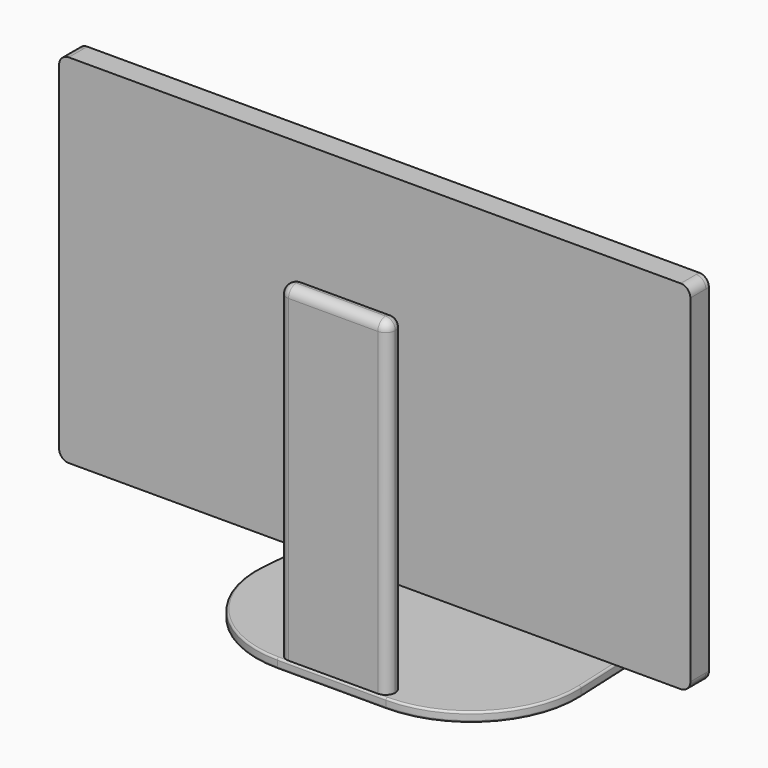
from build123d import *

# Parameters (mm, degrees)
F1_DEPTH    = 5
F2_R        = 1
F3_W        = 56.1862232486
F3_H        = 10
F4_DEPTH    = 170
F5_T1_DEPTH = 170
F6_T1_DEPTH = 170
F8_DEPTH    = 16
F9_R        = 4.99999
F11_DEPTH   = 10
F12_W       = 24
F12_H       = 13.9404982328
F13_DEPTH   = 10
F14_R       = 5
F15_R       = 5
F16_W       = 316.6455233097
F16_H       = 174.8104447126
F17_DEPTH   = 2
F18_W       = 15
F18_H       = 2
F19_DEPTH   = 0.5
F20_R       = 5
F21_R       = 5


# Not quite as in the source:
# - a fillet or chamfer that OpenCascade refuses, or shapes differently, is made with other operations: its cross-section is extruded or revolved along the edge and cut away or added
# - a fillet or chamfer is up to 0.001 mm smaller than in the source, because OpenCascade refuses the exact size


with BuildPart() as f1:
    # F0 (on Top) → F1 (new body)
    with BuildSketch(Plane.XY):
        with BuildLine():
            Line((23.2672947912, 89.7089094173), (-23.969883312, 89.7089094173))
            ThreePointArc((-23.969883312, 89.7089094173), (-61.030315745, 75.3478605341), (-78.737050658, 39.7643402492))
            Line((-78.737050658, 39.7643402492), (-84.7743571616, -25.63981354))
            ThreePointArc((-84.7743571616, -25.63981354), (-70.6461409325, -67.7556768049), (-30.0071898156, -85.6952443719))
            Line((-30.0071898156, -85.6952443719), (26.1790334329, -85.6952443719))
            ThreePointArc((26.1790334329, -85.6952443719), (65.9253366057, -68.7114433416), (81.1246105138, -28.2491128847))
            Line((81.1246105138, -28.2491128847), (78.2128718721, 37.1550409045))
            ThreePointArc((78.2128718721, 37.1550409045), (61.2834937609, 74.45521259), (23.2672947912, 89.7089094173))
        make_face()
    extrude(amount=F1_DEPTH)

    # F2
    f2_edges = [f1.edges().sort_by_distance(p)[0] for p in [
        (79.668741, 4.452964, 0),
        (61.283494, 74.455213, 0),
        (-0.351294, 89.708909, 0),
        (-61.030316, 75.347861, 0),
        (-81.755704, 7.062263, 0),
        (-70.646141, -67.755677, 0),
        (-1.914078, -85.695244, 0),
        (65.925337, -68.711443, 0),
        (79.668741, 4.452964, 5),
        (61.283494, 74.455213, 5),
        (-0.351294, 89.708909, 5),
        (-61.030316, 75.347861, 5),
        (-81.755704, 7.062263, 5),
        (-70.646141, -67.755677, 5),
        (-1.914078, -85.695244, 5),
        (65.925337, -68.711443, 5),
    ]]
    fillet(f2_edges, radius=F2_R)

    # F3 (on face) → F4 (join)
    with BuildSketch(Plane.XY.offset(5)):
        with Locations((-1.9140781913, -79.6952443719)):
            Rectangle(F3_W, F3_H)
    extrude(amount=F4_DEPTH)

    # F5: fillet of radius 5 on 1 edges, made by hand

    # F5_s2 → F5_t1 (cut)
    with BuildSketch(Plane.XY.offset(5)):
        with BuildLine():
            ThreePointArc((26.1790334329, -79.6952443719), (24.7145673389, -83.2307782778), (21.1790334329, -84.6952443719))
            Line((21.1790334329, -84.6952443719), (21.1790334329, -84.7952443719))
            Line((21.1790334329, -84.7952443719), (26.2790334329, -84.7952443719))
            Line((26.2790334329, -84.7952443719), (26.2790334329, -79.6952443719))
            Line((26.2790334329, -79.6952443719), (26.1790334329, -79.6952443719))
        make_face()
    extrude(amount=F5_T1_DEPTH, mode=Mode.SUBTRACT)

    # F6: fillet of radius 5 on 3 edges, made by hand

    # F6_s2 → F6_t1 (cut)
    with BuildSketch(Plane.XY.offset(5)):
        with BuildLine():
            ThreePointArc((21.1790334329, -74.6952443719), (24.7145673389, -76.159710466), (26.1790334329, -79.6952443719))
            Line((26.1790334329, -79.6952443719), (26.2790334329, -79.6952443719))
            Line((26.2790334329, -79.6952443719), (26.2790334329, -74.5952443719))
            Line((26.2790334329, -74.5952443719), (21.1790334329, -74.5952443719))
            Line((21.1790334329, -74.5952443719), (21.1790334329, -74.6952443719))
        make_face()
        with BuildLine():
            ThreePointArc((-25.0071898156, -74.6952443719), (-28.5427237216, -76.159710466), (-30.0071898156, -79.6952443719))
            Line((-30.0071898156, -79.6952443719), (-30.1071898156, -79.6952443719))
            Line((-30.1071898156, -79.6952443719), (-30.1071898156, -74.5952443719))
            Line((-30.1071898156, -74.5952443719), (-25.0071898156, -74.5952443719))
            Line((-25.0071898156, -74.5952443719), (-25.0071898156, -74.6952443719))
        make_face()
        with BuildLine():
            ThreePointArc((-30.0071898156, -79.6952443719), (-28.5427237216, -83.2307782778), (-25.0071898156, -84.6952443719))
            Line((-25.0071898156, -84.6952443719), (-25.0071898156, -84.7952443719))
            Line((-25.0071898156, -84.7952443719), (-30.1071898156, -84.7952443719))
            Line((-30.1071898156, -84.7952443719), (-30.1071898156, -79.6952443719))
            Line((-30.1071898156, -79.6952443719), (-30.0071898156, -79.6952443719))
        make_face()
    extrude(amount=F6_T1_DEPTH, mode=Mode.SUBTRACT)

    # F7 (on face) → F8 (join)
    with BuildSketch(Plane(origin=(0, -74.6952443719, 0), x_dir=(-1, 0, 0), z_dir=(0, 1, 0))):
        Polygon((13.9140781913, 140.0128751993), (1.9140781913, 140.0128751993), (-10.0859218087, 140.0128751993), (-10.0859218087, 126.0723769665), (13.9140781913, 126.0723769665), align=None)
    extrude(amount=F8_DEPTH)

    # F9 (radius 5 in the source; OpenCascade refuses exactly that, so slightly less here)
    f9_edges = [f1.edges().sort_by_distance(p)[0] for p in [
        (-1.914078, -74.695244, 175),
        (-28.542724, -76.15971, 175),
        (24.714567, -76.15971, 175),
        (24.714567, -83.230778, 175),
        (-1.914078, -84.695244, 175),
        (-28.542724, -83.230778, 175),
    ]]
    fillet(f9_edges, radius=F9_R)

    # F20
    f20_edges = [f1.edges().sort_by_distance(p)[0] for p in [
        (-13.914078, -66.695244, 140.012875),
    ]]
    fillet(f20_edges, radius=F20_R)

    # F21
    f21_edges = [f1.edges().sort_by_distance(p)[0] for p in [
        (-13.914078, -66.695244, 126.072377),
        (10.085922, -66.695244, 140.012875),
        (10.085922, -66.695244, 126.072377),
    ]]
    fillet(f21_edges, radius=F21_R)


with BuildPart() as f11:
    # F10 (on face) → F11 (new body)
    with BuildSketch(Plane(origin=(0, -58.6952443719, 0), x_dir=(-1, 0, 0), z_dir=(0, 1, 0))):
        Polygon((164.5585149527, 225.5081981421), (1.9140781913, 225.5081981421), (-162.087008357, 225.5081981421), (-162.087008357, 40.6977534294), (-160.0567102432, 40.6977534294), (164.5585149527, 40.6977534294), align=None)
        Polygon((-10.0859218087, 140.0128751993), (1.9140781913, 140.0128751993), (13.9140781913, 140.0128751993), (13.9140781913, 126.0723769665), (-10.0859218087, 126.0723769665), align=None, mode=Mode.SUBTRACT)
    extrude(amount=F11_DEPTH)

    # F14
    f14_edges = [f11.edges().sort_by_distance(p)[0] for p in [
        (162.087008, -53.695244, 225.508198),
    ]]
    fillet(f14_edges, radius=F14_R)

    # F15
    f15_edges = [f11.edges().sort_by_distance(p)[0] for p in [
        (-164.558515, -53.695244, 225.508198),
        (-164.558515, -53.695244, 40.697753),
        (162.087008, -53.695244, 40.697753),
    ]]
    fillet(f15_edges, radius=F15_R)

    # F16 (on face) → F17 (join)
    with BuildSketch(Plane(origin=(0, -48.6952443719, 0), x_dir=(-1, 0, 0), z_dir=(0, 1, 0))):
        with BuildLine():
            ThreePointArc((164.5585149527, 220.5081981421), (163.0940488586, 224.043732048), (159.5585149527, 225.5081981421))
            Line((159.5585149527, 225.5081981421), (-157.087008357, 225.5081981421))
            ThreePointArc((-157.087008357, 225.5081981421), (-160.622542263, 224.043732048), (-162.087008357, 220.5081981421))
            Line((-162.087008357, 220.5081981421), (-162.087008357, 45.6977534294))
            ThreePointArc((-162.087008357, 45.6977534294), (-160.622542263, 42.1622195235), (-157.087008357, 40.6977534294))
            Line((-157.087008357, 40.6977534294), (159.5585149527, 40.6977534294))
            ThreePointArc((159.5585149527, 40.6977534294), (163.0940488586, 42.1622195235), (164.5585149527, 45.6977534294))
            Line((164.5585149527, 45.6977534294), (164.5585149527, 220.5081981421))
        make_face()
        with Locations((1.2357532978, 133.1029757857)):
            Rectangle(F16_W, F16_H, mode=Mode.SUBTRACT)
    extrude(amount=F17_DEPTH)

    # F18 (on face) → F19 (join)
    with BuildSketch(Plane(origin=(0, -46.6952443719, 0), x_dir=(-1, 0, 0), z_dir=(0, 1, 0))):
        with Locations((97.4538546801, 43.1977534294)):
            Rectangle(F18_W, F18_H)
        with Locations((114.5963103771, 43.1977534294)):
            Rectangle(F18_W, F18_H)
        Polygon((139.0963103771, 42.1977534294), (139.0963103771, 44.1977534294), (129.0963103771, 44.1977534294), (124.0963103771, 44.1977534294), (124.0963103771, 42.1977534294), (130.4579966664, 42.1977534294), align=None)
    extrude(amount=F19_DEPTH)


with BuildPart() as f13:
    # F12 (on face) → F13 (new body)
    with BuildSketch(Plane(origin=(0, -58.6952443719, 0), x_dir=(-1, 0, 0), z_dir=(0, 1, 0))):
        with Locations((1.9140781913, 133.0426260829)):
            Rectangle(F12_W, F12_H)
    extrude(amount=F13_DEPTH)


solid = Compound([f1.part, f11.part, f13.part])
